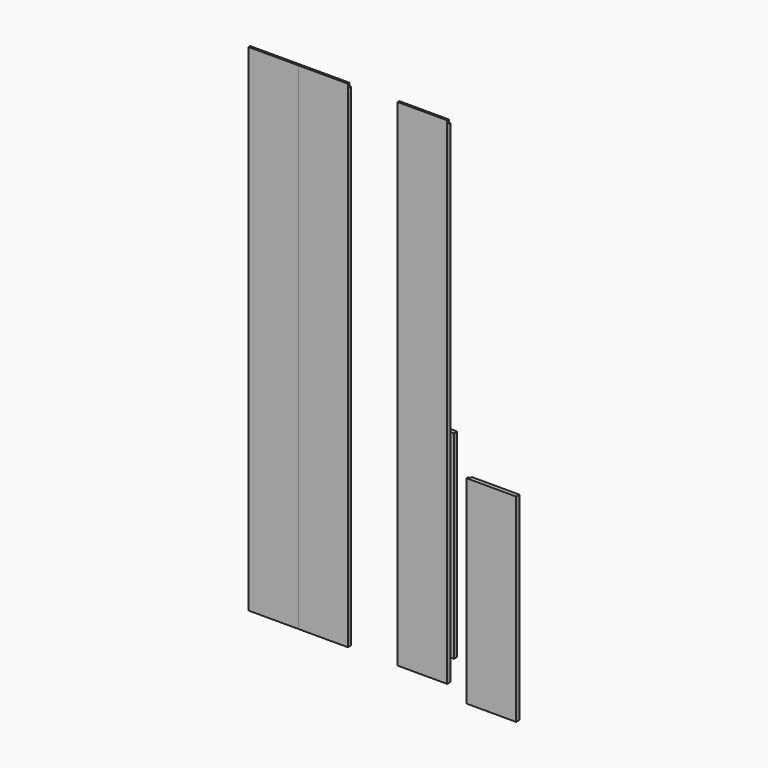
from build123d import *

# Parameters (mm, degrees)
F1_DEPTH  = 1524
F3_DEPTH  = 609.6
F6_W      = 133.35
F6_H      = 12.7
F7_DEPTH  = 6.35
F8_W      = 146.05
F8_H      = 12.7
F9_DEPTH  = 6.35
F12_W     = 139.7
F12_H     = 12.7
F13_DEPTH = 609.6


with BuildPart() as f1:
    # F0 (on Top) → F1 (new body)
    with BuildSketch(Plane.XY):
        Polygon((0, 6.35), (0, 0), (152.4, 0), (152.4, 12.7), (6.35, 12.7), (6.35, 6.35), align=None)
    extrude(amount=F1_DEPTH)

    # F6 (on face) → F7 (cut)
    with BuildSketch(Plane(origin=(0, 12.7, 0), x_dir=(-1, 0, 0), z_dir=(0, 1, 0))):
        with Locations((-73.025, 31.75)):
            Rectangle(F6_W, F6_H)
    extrude(amount=-F7_DEPTH, mode=Mode.SUBTRACT)

    # F8 (on face) → F9 (cut)
    with BuildSketch(Plane(origin=(0, 12.7, 0), x_dir=(-1, 0, 0), z_dir=(0, 1, 0))):
        with Locations((-79.375, 1517.65)):
            Rectangle(F8_W, F8_H)
    extrude(amount=-F9_DEPTH, mode=Mode.SUBTRACT)


with BuildPart() as f3:
    # F2 (on Top) → F3 (new body)
    with BuildSketch(Plane.XY):
        Polygon((-52.4232854942, -44.5139594376), (-52.4232854942, -50.8639594376), (99.9767145058, -50.8639594376), (99.9767145058, -38.1639594376), (-46.0732854942, -38.1639594376), (-46.0732854942, -44.5139594376), align=None)
    extrude(amount=F3_DEPTH)


with BuildPart() as f3_1:
    # F4: moved
    add(f3.part.moved(Location((152.4, 0, 0))))


with BuildPart() as f3_2:
    # F5: moved
    add(f3_1.part.moved(Location((152.4, 0, 0))))


with BuildPart() as f10_1:
    # F10: copy of F1
    add(f1.part.moved(Location((-304.8, 0, 0))))


with BuildPart() as f11_1:
    # F11: instance of F10_1
    add(f10_1.part.mirror(Plane(origin=(-304.8, 3.175, 762), x_dir=(0, -1, 0), z_dir=(-1, 0, 0))))


with BuildPart() as f13:
    # F12 (on Top) → F13 (new body)
    with BuildSketch(Plane.XY):
        with Locations((13.8991219759, 118.2391904384)):
            Rectangle(F12_W, F12_H)
    extrude(amount=F13_DEPTH)


solid = Compound([f1.part, f3_2.part, f10_1.part, f11_1.part, f13.part])
